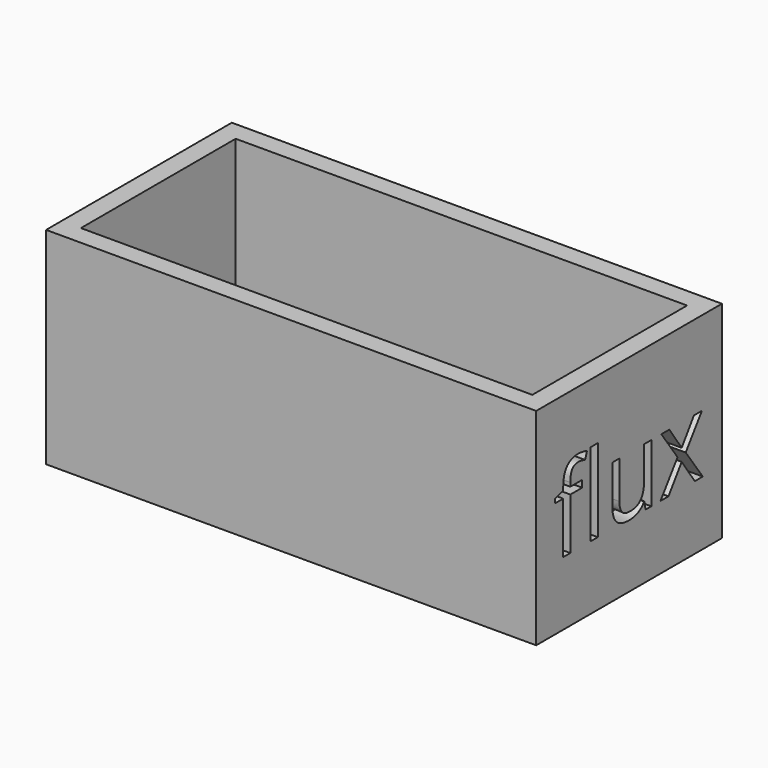
from build123d import *

# Parameters (mm, degrees)
F0_W         = 75.9999984503
F0_H         = 35.9999984503
F0_W_2       = 70
F0_H_2       = 30
F1_DEPTH     = 15
F2_W         = 75.9999984503
F2_H         = 35.9999984503
F3_DEPTH     = 2
F4_TEXT_SIZE = 16.9073617471
F5_DEPTH     = 5


# Not quite as in the source:
# - Text() gives the source's letters only with a copy of the font that has no kerning and outlines rounded to 1/6400 em; it was checked with that copy


with BuildPart() as f1:
    # F0 (on Top) → F1 (new body, symmetric)
    with BuildSketch(Plane.XY):
        Rectangle(F0_W, F0_H)
        Rectangle(F0_W_2, F0_H_2, mode=Mode.SUBTRACT)
    extrude(amount=F1_DEPTH, both=True)

    # F2 (on face) → F3 (join)
    with BuildSketch(Plane(origin=(0, 0, -15), x_dir=(1, 0, 0), z_dir=(0, 0, -1))):
        Rectangle(F2_W, F2_H)
    extrude(amount=F3_DEPTH)

    # F4 (on face) → F5 (cut)
    with BuildSketch(Plane.YZ.offset(37.9999992251)):
        with Locations((-14.615471357, -7.0876122243)):
            Text('flux', F4_TEXT_SIZE, font='Open Sans', text_align=(TextAlign.LEFT, TextAlign.BOTTOM))
    extrude(amount=-F5_DEPTH, mode=Mode.SUBTRACT)


solid = f1.part
